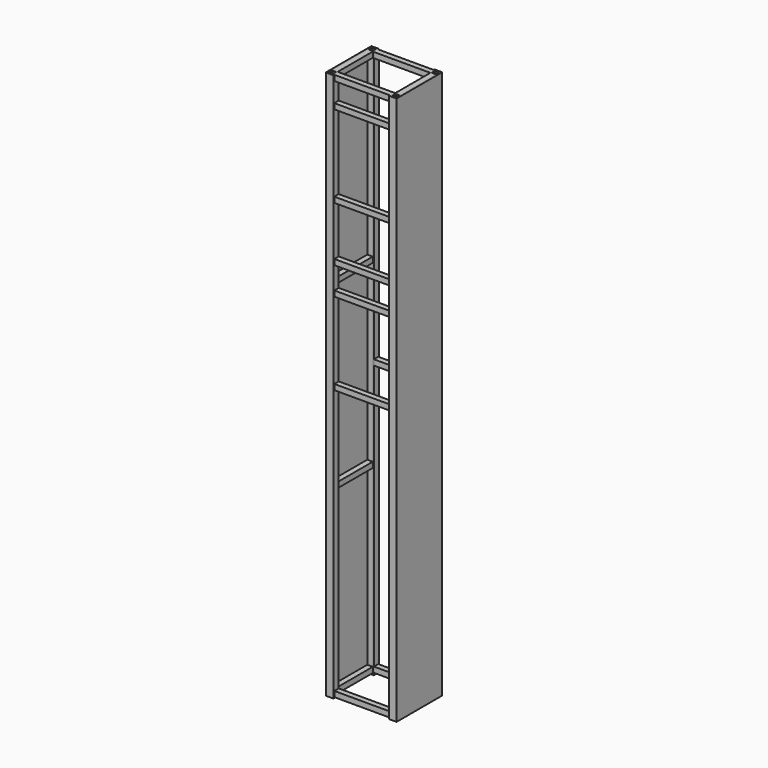
from build123d import *

# Parameters (mm, degrees)
F0_W     = 20
F0_H     = 20
F0_W_2   = 14
F0_H_2   = 14
F1_DEPTH = 2000
F3_DEPTH = 2000
F4_W     = 20
F4_H     = 20
F4_W_2   = 14
F4_H_2   = 14
F5_DEPTH = 210
F6_W     = 20
F6_H     = 20
F6_W_2   = 14
F6_H_2   = 14
F7_DEPTH = 160
F8_W     = 20
F8_H     = 20
F8_W_2   = 14
F8_H_2   = 14
F9_DEPTH = 210


# Not quite as in the source:
# - a feature names something its author has since deleted; it is built from what else it names


with BuildPart() as f1:
    # F0 (on Top) → F1 (new body)
    with BuildSketch(Plane.XY):
        with Locations((10, 190)):
            Rectangle(F0_W, F0_H)
        with Locations((10, 190)):
            Rectangle(F0_W_2, F0_H_2, mode=Mode.SUBTRACT)
    extrude(amount=F1_DEPTH)


with BuildPart() as f1b:
    # F0 (on Top) → F1, piece 2 (new body)
    with BuildSketch(Plane.XY):
        with Locations((240, 190)):
            Rectangle(F0_W, F0_H)
        with Locations((240, 190)):
            Rectangle(F0_W_2, F0_H_2, mode=Mode.SUBTRACT)
    extrude(amount=F1_DEPTH)


with BuildPart() as f1c:
    # F0 (on Top) → F1, piece 3 (new body)
    with BuildSketch(Plane.XY):
        with Locations((240, 10)):
            Rectangle(F0_W, F0_H)
        with Locations((240, 10)):
            Rectangle(F0_W_2, F0_H_2, mode=Mode.SUBTRACT)
    extrude(amount=F1_DEPTH)


with BuildPart() as f1d:
    # F0 (on Top) → F1, piece 4 (new body)
    with BuildSketch(Plane.XY):
        with Locations((10, 10)):
            Rectangle(F0_W, F0_H)
        with Locations((10, 10)):
            Rectangle(F0_W_2, F0_H_2, mode=Mode.SUBTRACT)
    extrude(amount=F1_DEPTH)


with BuildPart() as f3:
    # F2 (on Top) → F3 (new body)
    with BuildSketch(Plane.XY):
        Polygon((20.0002528727, 0), (0, 0), (0, 200.0347077847), (20.113453269, 200.0347077847), (20.113453269, 179.9583435059), (24.113453269, 179.9583435059), (24, 204), (-4, 204), (-4, -4), (24.0002528727, -4), (24.0002528727, 20), (20.0002528727, 20), align=None)
    extrude(amount=F3_DEPTH)


with BuildPart() as f3b:
    # F2 (on Top) → F3, piece 2 (new body)
    with BuildSketch(Plane.XY):
        Polygon((229.9997471273, 20), (225.9997471273, 20), (225.9997471273, -4), (254, -4), (254, 204), (226, 204), (226.0000001659, 179.8393327155), (230, 179.838180542), (230, 199.9974697828), (250, 199.9974697828), (250, 0), (229.9997471273, 0), align=None)
    extrude(amount=F3_DEPTH)


with BuildPart() as f5:
    # F4 (on face) → F5 (new body)
    with BuildSketch(Plane.YZ.offset(20)):
        with Locations((10, 1990)):
            Rectangle(F4_W, F4_H)
        with Locations((10, 1990)):
            Rectangle(F4_W_2, F4_H_2, mode=Mode.SUBTRACT)
    extrude(amount=F5_DEPTH)


with BuildPart() as f5b:
    # F4 (on face) → F5, piece 2 (new body)
    with BuildSketch(Plane.YZ.offset(20)):
        with Locations((10, 1899)):
            Rectangle(F4_W, F4_H)
        with Locations((10, 1899)):
            Rectangle(F4_W_2, F4_H_2, mode=Mode.SUBTRACT)
    extrude(amount=F5_DEPTH)


with BuildPart() as f5c:
    # F4 (on face) → F5, piece 3 (new body)
    with BuildSketch(Plane.YZ.offset(20)):
        with Locations((10, 1599)):
            Rectangle(F4_W, F4_H)
        with Locations((10, 1599)):
            Rectangle(F4_W_2, F4_H_2, mode=Mode.SUBTRACT)
    extrude(amount=F5_DEPTH)


with BuildPart() as f5d:
    # F4 (on face) → F5, piece 4 (new body)
    with BuildSketch(Plane.YZ.offset(20)):
        with Locations((10, 1399)):
            Rectangle(F4_W, F4_H)
        with Locations((10, 1399)):
            Rectangle(F4_W_2, F4_H_2, mode=Mode.SUBTRACT)
    extrude(amount=F5_DEPTH)


with BuildPart() as f5e:
    # F4 (on face) → F5, piece 5 (new body)
    with BuildSketch(Plane.YZ.offset(20)):
        with Locations((10, 1298)):
            Rectangle(F4_W, F4_H)
        with Locations((10, 1298)):
            Rectangle(F4_W_2, F4_H_2, mode=Mode.SUBTRACT)
    extrude(amount=F5_DEPTH)


with BuildPart() as f5f:
    # F4 (on face) → F5, piece 6 (new body)
    with BuildSketch(Plane.YZ.offset(20)):
        with Locations((10, 998)):
            Rectangle(F4_W, F4_H)
        with Locations((10, 998)):
            Rectangle(F4_W_2, F4_H_2, mode=Mode.SUBTRACT)
    extrude(amount=F5_DEPTH)


with BuildPart() as f5g:
    # F4 (on face) → F5, piece 7 (new body)
    with BuildSketch(Plane.YZ.offset(20)):
        with Locations((10, 13)):
            Rectangle(F4_W, F4_H)
        with Locations((10, 13)):
            Rectangle(F4_W_2, F4_H_2, mode=Mode.SUBTRACT)
    extrude(amount=F5_DEPTH)


with BuildPart() as f7:
    # F6 (on face) → F7 (new body)
    with BuildSketch(Plane(origin=(0, 20, 0), x_dir=(-1, 0, 0), z_dir=(0, 1, 0))):
        with Locations((-10, 1990)):
            Rectangle(F6_W, F6_H)
        with Locations((-10, 1990)):
            Rectangle(F6_W_2, F6_H_2, mode=Mode.SUBTRACT)
    extrude(amount=F7_DEPTH)


with BuildPart() as f7b:
    # F6 (on face) → F7, piece 2 (new body)
    with BuildSketch(Plane(origin=(0, 20, 0), x_dir=(-1, 0, 0), z_dir=(0, 1, 0))):
        with Locations((-240, 1990)):
            Rectangle(F6_W, F6_H)
        with Locations((-240, 1990)):
            Rectangle(F6_W_2, F6_H_2, mode=Mode.SUBTRACT)
    extrude(amount=F7_DEPTH)


with BuildPart() as f7c:
    # F6 (on face) → F7, piece 3 (new body)
    with BuildSketch(Plane(origin=(0, 20, 0), x_dir=(-1, 0, 0), z_dir=(0, 1, 0))):
        with Locations((-10, 1332)):
            Rectangle(F6_W, F6_H)
        with Locations((-10, 1332)):
            Rectangle(F6_W_2, F6_H_2, mode=Mode.SUBTRACT)
    extrude(amount=F7_DEPTH)


with BuildPart() as f7d:
    # F6 (on face) → F7, piece 4 (new body)
    with BuildSketch(Plane(origin=(0, 20, 0), x_dir=(-1, 0, 0), z_dir=(0, 1, 0))):
        with Locations((-240, 1332)):
            Rectangle(F6_W, F6_H)
        with Locations((-240, 1332)):
            Rectangle(F6_W_2, F6_H_2, mode=Mode.SUBTRACT)
    extrude(amount=F7_DEPTH)


with BuildPart() as f7e:
    # F6 (on face) → F7, piece 5 (new body)
    with BuildSketch(Plane(origin=(0, 20, 0), x_dir=(-1, 0, 0), z_dir=(0, 1, 0))):
        with Locations((-10, 674)):
            Rectangle(F6_W, F6_H)
        with Locations((-10, 674)):
            Rectangle(F6_W_2, F6_H_2, mode=Mode.SUBTRACT)
    extrude(amount=F7_DEPTH)


with BuildPart() as f7f:
    # F6 (on face) → F7, piece 6 (new body)
    with BuildSketch(Plane(origin=(0, 20, 0), x_dir=(-1, 0, 0), z_dir=(0, 1, 0))):
        with Locations((-240, 674)):
            Rectangle(F6_W, F6_H)
        with Locations((-240, 674)):
            Rectangle(F6_W_2, F6_H_2, mode=Mode.SUBTRACT)
    extrude(amount=F7_DEPTH)


with BuildPart() as f7g:
    # F6 (on face) → F7, piece 7 (new body)
    with BuildSketch(Plane(origin=(0, 20, 0), x_dir=(-1, 0, 0), z_dir=(0, 1, 0))):
        with Locations((-10, 16)):
            Rectangle(F6_W, F6_H)
        with Locations((-10, 16)):
            Rectangle(F6_W_2, F6_H_2, mode=Mode.SUBTRACT)
    extrude(amount=F7_DEPTH)


with BuildPart() as f7h:
    # F6 (on face) → F7, piece 8 (new body)
    with BuildSketch(Plane(origin=(0, 20, 0), x_dir=(-1, 0, 0), z_dir=(0, 1, 0))):
        with Locations((-240, 16)):
            Rectangle(F6_W, F6_H)
        with Locations((-240, 16)):
            Rectangle(F6_W_2, F6_H_2, mode=Mode.SUBTRACT)
    extrude(amount=F7_DEPTH)


with BuildPart() as f9:
    # F8 (on face) → F9 (new body)
    with BuildSketch(Plane.YZ.offset(20)):
        with Locations((190, 1990)):
            Rectangle(F8_W, F8_H)
        with Locations((190, 1990)):
            Rectangle(F8_W_2, F8_H_2, mode=Mode.SUBTRACT)
    extrude(amount=F9_DEPTH)


with BuildPart() as f9b:
    # F8 (on face) → F9, piece 2 (new body)
    with BuildSketch(Plane.YZ.offset(20)):
        with Locations((190, 1004)):
            Rectangle(F8_W, F8_H)
        with Locations((190, 1004)):
            Rectangle(F8_W_2, F8_H_2, mode=Mode.SUBTRACT)
    extrude(amount=F9_DEPTH)


with BuildPart() as f9c:
    # F8 (on face) → F9, piece 3 (new body)
    with BuildSketch(Plane.YZ.offset(20)):
        with Locations((190, 18)):
            Rectangle(F8_W, F8_H)
        with Locations((190, 18)):
            Rectangle(F8_W_2, F8_H_2, mode=Mode.SUBTRACT)
    extrude(amount=F9_DEPTH)


solid = Compound([f1.part, f1b.part, f1c.part, f1d.part, f3.part, f3b.part, f5.part, f5b.part, f5c.part, f5d.part, f5e.part, f5f.part, f5g.part, f7.part, f7b.part, f7c.part, f7d.part, f7e.part, f7f.part, f7g.part, f7h.part, f9.part, f9b.part, f9c.part])
